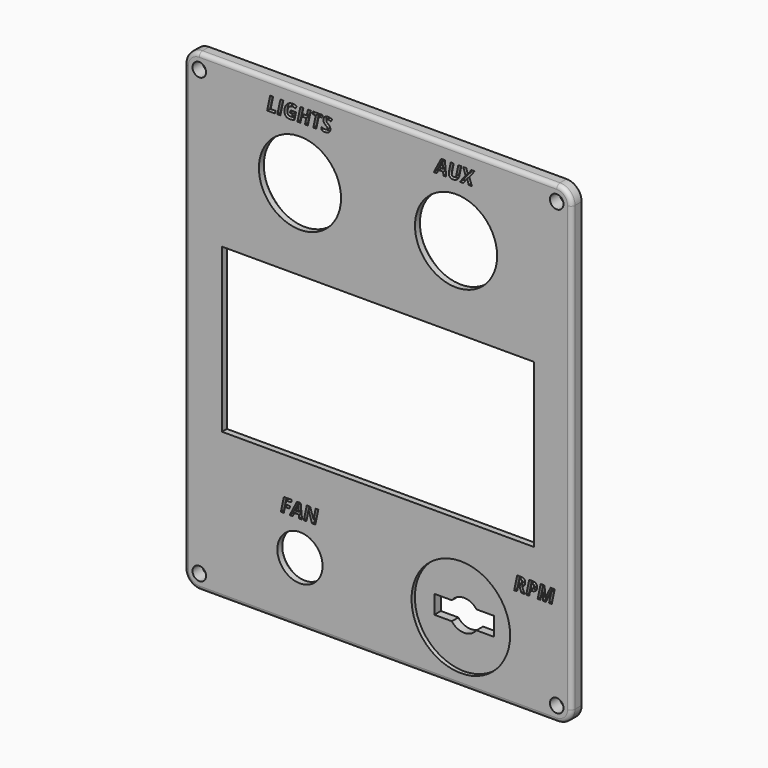
from build123d import *

# Parameters (mm, degrees)
F0_R         = 5.5
F0_W         = 75.946
F0_H         = 39.675
F0_R_2       = 10
F1_DEPTH     = 3
F2_SIZE      = 1.5
F3_R         = 12
F4_DEPTH     = 1
F5_D         = 3.3
F6_R         = 1
F7_TEXT_SIZE = 4.816013312
F8_DEPTH     = 1


# Not quite as in the source:
# - Text() gives the source's letters only with a copy of the font that has no kerning and outlines rounded to 1/6400 em; it was checked with that copy


with BuildPart() as f1:
    # F0 (on Front) → F1 (new body)
    with BuildSketch(Plane.XZ):
        with BuildLine():
            ThreePointArc((47.165, 53.9825), (46.0930108191, 56.5705108191), (43.505, 57.6425))
            Line((43.505, 57.6425), (-43.505, 57.6425))
            ThreePointArc((-43.505, 57.6425), (-46.0930108191, 56.5705108191), (-47.165, 53.9825))
            Line((-47.165, 53.9825), (-47.165, -53.9825))
            ThreePointArc((-47.165, -53.9825), (-46.0930108191, -56.5705108191), (-43.505, -57.6425))
            Line((-43.505, -57.6425), (43.505, -57.6425))
            ThreePointArc((43.505, -57.6425), (46.0930108191, -56.5705108191), (47.165, -53.9825))
            Line((47.165, -53.9825), (47.165, 53.9825))
        make_face()
        with Locations((-19, -42.6425)):
            Circle(F0_R, mode=Mode.SUBTRACT)
        with BuildLine():
            Line((23.165, -40.3925), (27.415, -40.3925))
            Line((27.415, -40.3925), (27.415, -44.8925))
            Line((27.415, -44.8925), (23.165, -44.8925))
            ThreePointArc((23.165, -44.8925), (20.165, -46.3925), (17.165, -44.8925))
            Line((17.165, -44.8925), (12.915, -44.8925))
            Line((12.915, -44.8925), (12.915, -40.3925))
            Line((12.915, -40.3925), (17.165, -40.3925))
            ThreePointArc((17.165, -40.3925), (20.165, -38.8925), (23.165, -40.3925))
        make_face(mode=Mode.SUBTRACT)
        with Locations((0, -1.97)):
            Rectangle(F0_W, F0_H, mode=Mode.SUBTRACT)
        with Locations((-19, 37.6425)):
            Circle(F0_R_2, mode=Mode.SUBTRACT)
        with Locations((19, 37.6425)):
            Circle(F0_R_2, mode=Mode.SUBTRACT)
    extrude(amount=F1_DEPTH)

    # F2
    f2_edges = [f1.edges().sort_by_distance(p)[0] for p in [
        (0, 0, 17.8675),
        (-37.973, 0, -1.97),
        (0, 0, -21.8075),
        (37.973, 0, -1.97),
        (9, 0, 37.6425),
        (-29, 0, 37.6425),
        (-24.5, 0, -42.6425),
    ]]
    chamfer(f2_edges, length=F2_SIZE)

    # F3 (on face) → F4 (cut)
    with BuildSketch(Plane.XZ.offset(3)):
        with Locations((20.165, -42.6425)):
            Circle(F3_R)
    extrude(amount=-F4_DEPTH, mode=Mode.SUBTRACT)

    # F5 (through all)
    with Locations(Plane(origin=(0, 0, 0), x_dir=(1, 0, 0), z_dir=(0, 1, 0))):
        with Locations((-43.505, -53.9825), (43.505, -53.9825), (-43.505, 53.9825), (43.505, 53.9825)):
            Hole(F5_D / 2)

    # F6
    f6_edges = [f1.edges().sort_by_distance(p)[0] for p in [
        (0, -3, -57.6425),
        (-46.093011, -3, -56.570511),
        (-47.165, -3, 0),
        (-46.093011, -3, 56.570511),
        (0, -3, 57.6425),
        (46.093011, -3, 56.570511),
        (47.165, -3, 0),
        (46.093011, -3, -56.570511),
    ]]
    fillet(f6_edges, radius=F6_R)

    # F7 (on face) → F8 (cut)
    with BuildSketch(Plane.XZ.offset(3)):
        with Locations((-27.1093386652, 50.5987352077)):
            Text('LIGHTS', F7_TEXT_SIZE, font='Open Sans', font_style=FontStyle.BOLDITALIC, text_align=(TextAlign.LEFT, TextAlign.BOTTOM))
        with Locations((13.8762133373, 50.5987352077)):
            Text('AUX', F7_TEXT_SIZE, font='Open Sans', font_style=FontStyle.BOLDITALIC, text_align=(TextAlign.LEFT, TextAlign.BOTTOM))
        with Locations((-23.7761307018, -34.3085664981)):
            Text('FAN', F7_TEXT_SIZE, font='Open Sans', font_style=FontStyle.BOLDITALIC, text_align=(TextAlign.LEFT, TextAlign.BOTTOM))
        with Locations((33.0265574157, -32.6427347409)):
            Text('RPM', F7_TEXT_SIZE, font='Open Sans', font_style=FontStyle.BOLDITALIC, text_align=(TextAlign.LEFT, TextAlign.BOTTOM))
    extrude(amount=-F8_DEPTH, mode=Mode.SUBTRACT)


solid = f1.part
